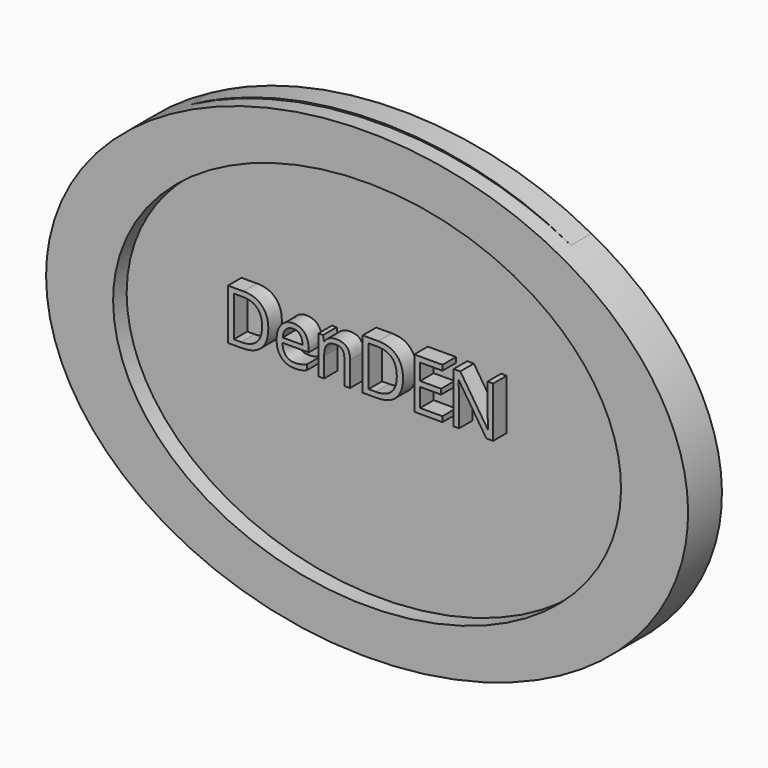
from build123d import *

# Parameters (mm, degrees)
F1_DEPTH     = 3.81
F2_TEXT_SIZE = 10.6170385455
F3_DEPTH     = 2.54
F5_DEPTH     = 6.35


# Not quite as in the source:
# - Text() gives the source's letters only with a copy of the font that has no kerning and outlines rounded to 1/6400 em; it was checked with that copy


with BuildPart() as f1:
    # F0 (on Front) → F1 (new body)
    with BuildSketch(Plane.XZ):
        with BuildLine():
            add(Edge.make_bspline(
                [(-47.625, 0), (-47.625, -60.4918744543), (23.8125, -30.2459372272), (95.25, 0), (23.8125, 30.2459372272), (-47.625, 60.4918744543), (-47.625, 0)],
                knots=[0, 0, 0, 2.0943951024, 2.0943951024, 4.1887902048, 4.1887902048, 6.2831853072, 6.2831853072, 6.2831853072], degree=2, weights=[1, 0.5, 1, 0.5, 1, 0.5, 1]))
        make_face()
    extrude(amount=F1_DEPTH)

    # F2 (on face) → F3 (join)
    with BuildSketch(Plane.XZ.offset(3.81)):
        with Locations((-21.91356197, 0)):
            Text('DenDEN', F2_TEXT_SIZE, font='Open Sans', text_align=(TextAlign.LEFT, TextAlign.BOTTOM))
    extrude(amount=F3_DEPTH)

    # F4 (on Front) → F5 (join)
    with BuildSketch(Plane.XZ):
        with BuildLine():
            add(Edge.make_bspline(
                [(-48.1588877738, 0), (-48.1588877738, -60.1206350757), (24.0794438869, -30.0603175379), (96.3177755475, 0), (24.0794438869, 30.0603175379), (-48.1588877738, 60.1206350757), (-48.1588877738, 0)],
                knots=[0, 0, 0, 2.0943951024, 2.0943951024, 4.1887902048, 4.1887902048, 6.2831853072, 6.2831853072, 6.2831853072], degree=2, weights=[1, 0.5, 1, 0.5, 1, 0.5, 1]))
        make_face()
        with BuildLine():
            add(Edge.make_bspline(
                [(-38.1, 0), (-38.1, -48.4362305319), (19.05, -24.2181152659), (76.2, 0), (19.05, 24.2181152659), (-38.1, 48.4362305319), (-38.1, 0)],
                knots=[0, 0, 0, 2.0943951024, 2.0943951024, 4.1887902048, 4.1887902048, 6.2831853072, 6.2831853072, 6.2831853072], degree=2, weights=[1, 0.5, 1, 0.5, 1, 0.5, 1]))
        make_face(mode=Mode.SUBTRACT)
    extrude(amount=F5_DEPTH)


solid = f1.part
